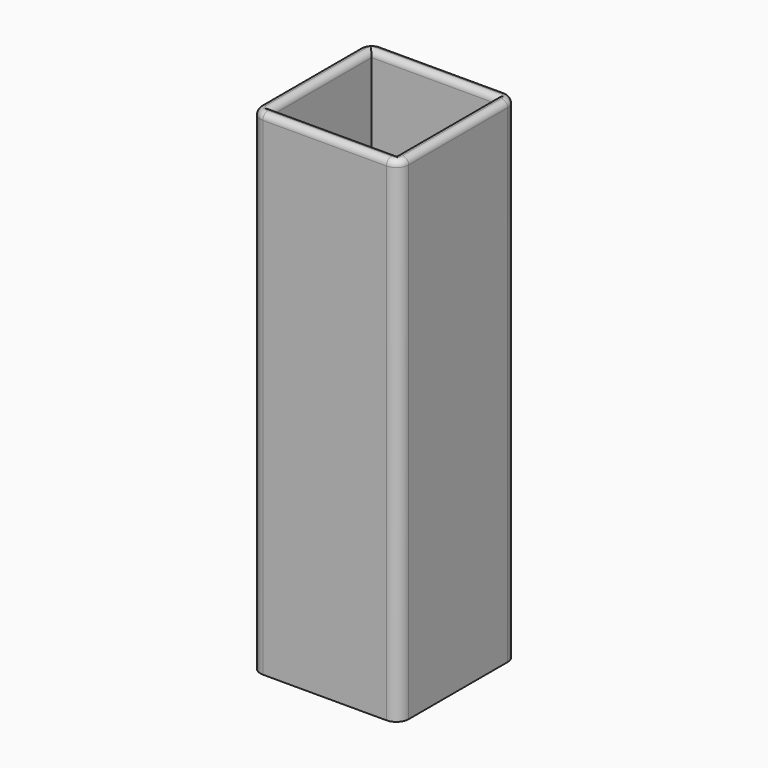
from build123d import *

# Parameters (mm, degrees)
F0_W         = 30
F0_H         = 30
F1_DEPTH     = 120
F2_R         = 1.5
F3_T1_DEPTH  = 30
F3_T3_DEPTH  = 30
F3_T6_ANGLE  = 90
F3_T8_ANGLE  = 90
F3_T10_ANGLE = 90
F3_T12_ANGLE = 90


# Not quite as in the source:
# - a fillet or chamfer that OpenCascade refuses, or shapes differently, is made with other operations: its cross-section is extruded or revolved along the edge and cut away or added


with BuildPart() as f1:
    # F0 (on Top) → F1 (new body)
    with BuildSketch(Plane.XY):
        with BuildLine():
            Line((33, 0), (3, 0))
            ThreePointArc((3, 0), (0.8786796564, -0.8786796564), (0, -3))
            Line((0, -3), (0, -33))
            ThreePointArc((0, -33), (0.8786796564, -35.1213203436), (3, -36))
            Line((3, -36), (33, -36))
            ThreePointArc((33, -36), (35.1213203436, -35.1213203436), (36, -33))
            Line((36, -33), (36, -3))
            ThreePointArc((36, -3), (35.1213203436, -0.8786796564), (33, 0))
        make_face()
        with Locations((18, -18)):
            Rectangle(F0_W, F0_H, mode=Mode.SUBTRACT)
    extrude(amount=F1_DEPTH)

    # F2
    f2_edges = [f1.edges().sort_by_distance(p)[0] for p in [
        (18, -33, 120),
        (3, -18, 120),
        (18, -3, 120),
        (33, -18, 120),
    ]]
    fillet(f2_edges, radius=F2_R)

    # F3: fillet of radius 1.5 on 4 edges, made by hand

    # F3_s2 → F3_t1 (cut)
    with BuildSketch(Plane.XZ.offset(3)):
        with BuildLine():
            ThreePointArc((34.5, 120), (35.5606601718, 119.5606601718), (36, 118.5))
            Line((36, 118.5), (36, 120))
            Line((36, 120), (34.5, 120))
        make_face()
        with BuildLine():
            ThreePointArc((1.5, 120), (0.4393398282, 119.5606601718), (0, 118.5))
            Line((0, 118.5), (0, 120))
            Line((0, 120), (1.5, 120))
        make_face()
    extrude(amount=F3_T1_DEPTH, mode=Mode.SUBTRACT)

    # F3_s4 → F3_t3 (cut)
    with BuildSketch(Plane.YZ.offset(3)):
        with BuildLine():
            ThreePointArc((-1.5, 120), (-0.4393398282, 119.5606601718), (0, 118.5))
            Line((0, 118.5), (0, 120))
            Line((0, 120), (-1.5, 120))
        make_face()
        with BuildLine():
            ThreePointArc((-34.5, 120), (-35.5606601718, 119.5606601718), (-36, 118.5))
            Line((-36, 118.5), (-36, 120))
            Line((-36, 120), (-34.5, 120))
        make_face()
    extrude(amount=F3_T3_DEPTH, mode=Mode.SUBTRACT)

    # F3_s5 → F3_t6 (revolve, cut)
    with BuildSketch(Plane.XZ.offset(3)):
        with BuildLine():
            ThreePointArc((34.5, 120), (35.5606601718, 119.5606601718), (36, 118.5))
            Line((36, 118.5), (36, 120))
            Line((36, 120), (34.5, 120))
        make_face()
    revolve(axis=Axis((33, -3, 120), (0, 0, 1)), revolution_arc=F3_T6_ANGLE, mode=Mode.SUBTRACT)

    # F3_s7 → F3_t8 (revolve, cut)
    with BuildSketch(Plane.YZ.offset(3)):
        with BuildLine():
            ThreePointArc((-1.5, 120), (-0.4393398282, 119.5606601718), (0, 118.5))
            Line((0, 118.5), (0, 120))
            Line((0, 120), (-1.5, 120))
        make_face()
    revolve(axis=Axis((3, -3, 120), (0, 0, 1)), revolution_arc=F3_T8_ANGLE, mode=Mode.SUBTRACT)

    # F3_s9 → F3_t10 (revolve, cut)
    with BuildSketch(Plane.XZ.offset(33)):
        with BuildLine():
            ThreePointArc((1.5, 120), (0.4393398282, 119.5606601718), (0, 118.5))
            Line((0, 118.5), (0, 120))
            Line((0, 120), (1.5, 120))
        make_face()
    revolve(axis=Axis((3, -33, 120), (0, 0, 1)), revolution_arc=F3_T10_ANGLE, mode=Mode.SUBTRACT)

    # F3_s11 → F3_t12 (revolve, cut)
    with BuildSketch(Plane.YZ.offset(33)):
        with BuildLine():
            ThreePointArc((-34.5, 120), (-35.5606601718, 119.5606601718), (-36, 118.5))
            Line((-36, 118.5), (-36, 120))
            Line((-36, 120), (-34.5, 120))
        make_face()
    revolve(axis=Axis((33, -33, 120), (0, 0, 1)), revolution_arc=F3_T12_ANGLE, mode=Mode.SUBTRACT)


solid = f1.part
